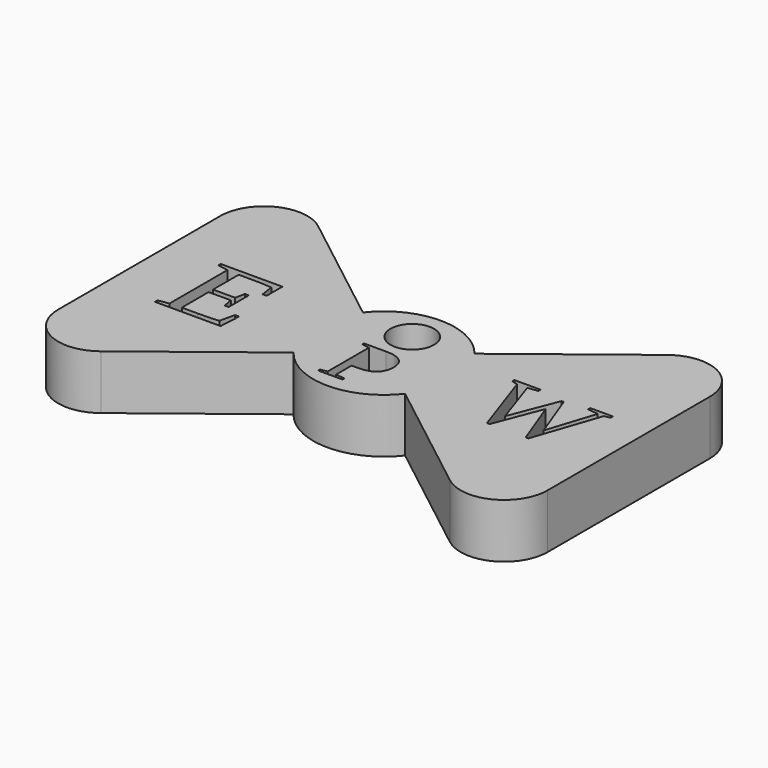
from build123d import *

# Parameters (mm, degrees)
F0_R     = 2
F1_DEPTH = 5


with BuildPart() as f1:
    # F0 (on Top) → F1 (new body)
    with BuildSketch(Plane.XY):
        with BuildLine():
            ThreePointArc((-3.8750014305, 0), (-4.2267672199, -2.1093164988), (-5.2439909973, -3.9903298027))
            Line((-5.2439909973, -3.9903298027), (5.6694109986, -12.4775612749))
            ThreePointArc((5.6694109986, -12.4775612749), (9.8825038634, -12.9132287637), (12.1249985695, -9.3200163929))
            Line((12.1249985695, -9.3200163929), (12.1249985695, 9.3200163929))
            ThreePointArc((12.1249985695, 9.3200163929), (9.8825038634, 12.9132287637), (5.6694109986, 12.4775612749))
            Line((5.6694109986, 12.4775612749), (-5.2439909973, 3.9903298027))
            ThreePointArc((-5.2439909973, 3.9903298027), (-4.2267672199, 2.1093164988), (-3.8750014305, 0))
        make_face()
        Polygon((8.0675292322, 2.2068999953), (6.0064843484, -3.8768709144), (5.756569483, -3.8768709144), (4.1200787681, 0.4710455388), (2.4399282273, -3.8768709144), (2.1900133619, -3.8768709144), (0.1018692759, 2.2068999953), (-0.449147837, 2.3288464056), (-0.449147837, 2.5787612709), (1.9596701426, 2.5787612709), (1.9596701426, 2.3288464056), (1.0337807317, 2.2068999953), (2.5347754353, -2.2388746883), (4.2329921109, 2.1361409672), (4.4437636841, 2.1361409672), (6.0817599103, -2.2388746883), (7.5119955856, 2.2068999953), (6.5288967477, 2.3288464056), (6.5288967477, 2.5787612709), (8.6170408338, 2.5787612709), (8.6170408338, 2.3288464056), align=None, mode=Mode.SUBTRACT)
        with BuildLine():
            ThreePointArc((-15.5059721811, 3.9903808286), (-16.8750014304, 3.23201e-05), (-15.5060118637, -3.9903298027))
            ThreePointArc((-15.5060118637, -3.9903298027), (-10.3750014305, -6.5), (-5.2439909973, -3.9903298027))
            ThreePointArc((-5.2439909973, -3.9903298027), (-4.2267672199, -2.1093164988), (-3.8750014305, 0))
            ThreePointArc((-3.8750014305, 0), (-4.2267672199, 2.1093164988), (-5.2439909973, 3.9903298027))
            ThreePointArc((-5.2439909973, 3.9903298027), (-10.3749691104, 6.4999999999), (-15.5059721811, 3.9903808286))
        make_face()
        with BuildLine():
            Line((-10.3772096263, -2.9674286779), (-10.9801440776, -2.9674286779))
            Line((-10.9801440776, -2.9674286779), (-10.9801440776, -4.7481291549))
            Line((-10.9801440776, -4.7481291549), (-10.1293933476, -4.8554310488))
            Line((-10.1293933476, -4.8554310488), (-10.1293933476, -5.0674800295))
            Line((-10.1293933476, -5.0674800295), (-12.385287926, -5.0674800295))
            Line((-12.385287926, -5.0674800295), (-12.385287926, -4.8554310488))
            Line((-12.385287926, -4.8554310488), (-11.7504183872, -4.7481291549))
            Line((-11.7504183872, -4.7481291549), (-11.7504183872, -0.0294006313))
            Line((-11.7504183872, -0.0294006313), (-12.4376614694, 0.0740690521))
            Line((-12.4376614694, 0.0740690521), (-12.4376614694, 0.2861180328))
            Line((-12.4376614694, 0.2861180328), (-10.4168091348, 0.2861180328))
            add(Edge.make_bspline(
                [(-10.4168091348, 0.2861180328), (-8.4534399575, 0.2861180328), (-8.4534399575, -1.2914752879)],
                knots=[0, 0, 0, 1, 1, 1], degree=2))
            add(Edge.make_bspline(
                [(-8.4534399575, -1.2914752879), (-8.4534399575, -2.1128457374), (-8.9503499185, -2.5401372077)],
                knots=[0, 0, 0, 1, 1, 1], degree=2))
            add(Edge.make_bspline(
                [(-8.9503499185, -2.5401372077), (-9.4472598794, -2.9674286779), (-10.3772096263, -2.9674286779)],
                knots=[0, 0, 0, 1, 1, 1], degree=2))
        make_face(mode=Mode.SUBTRACT)
        with Locations((-10.3750014305, 3.25)):
            Circle(F0_R, mode=Mode.SUBTRACT)
        with BuildLine():
            Line((-32.8750014305, 9.3202724501), (-32.8750014305, -9.3200163929))
            ThreePointArc((-32.8750014305, -9.3200163929), (-30.6325067245, -12.9132287637), (-26.4194138596, -12.4775612749))
            Line((-26.4194138596, -12.4775612749), (-15.5060118637, -3.9903298027))
            ThreePointArc((-15.5060118637, -3.9903298027), (-16.8750014304, 3.23201e-05), (-15.5059721811, 3.9903808286))
            Line((-15.5059721811, 3.9903808286), (-26.4193824591, 12.477792912))
            ThreePointArc((-26.4193824591, 12.477792912), (-30.6324888578, 12.9134935598), (-32.8750014305, 9.3202724501))
        make_face()
        with BuildLine():
            Line((-28.1915230864, -4.0461723693), (-28.1915230864, -3.7470318405))
            Line((-28.1915230864, -3.7470318405), (-27.2220194448, -3.5956595247))
            Line((-27.2220194448, -3.5956595247), (-27.2220194448, 3.0611182673))
            Line((-27.2220194448, 3.0611182673), (-28.1915230864, 3.2070844289))
            Line((-28.1915230864, 3.2070844289), (-28.1915230864, 3.5062249578))
            Line((-28.1915230864, 3.5062249578), (-22.5258735526, 3.5062249578))
            Line((-22.5258735526, 3.5062249578), (-22.5258735526, 1.6987674252))
            Line((-22.5258735526, 1.6987674252), (-22.8970961366, 1.6987674252))
            Line((-22.8970961366, 1.6987674252), (-23.0773012744, 2.9205582598))
            add(Edge.make_bspline(
                [(-23.0773012744, 2.9205582598), (-23.7080192569, 2.9980464691), (-24.9027793208, 2.9980464691)],
                knots=[0, 0, 0, 1, 1, 1], degree=2))
            Line((-24.9027793208, 2.9980464691), (-26.1353824636, 2.9980464691))
            Line((-26.1353824636, 2.9980464691), (-26.1353824636, 0.0480883625))
            Line((-26.1353824636, 0.0480883625), (-24.0972623546, 0.0480883625))
            Line((-24.0972623546, 0.0480883625), (-23.9224633709, 0.9491140518))
            Line((-23.9224633709, 0.9491140518), (-23.5620530952, 0.9491140518))
            Line((-23.5620530952, 0.9491140518), (-23.5620530952, -1.3719281237))
            Line((-23.5620530952, -1.3719281237), (-23.9224633709, -1.3719281237))
            Line((-23.9224633709, -1.3719281237), (-24.0972623546, -0.4582880748))
            Line((-24.0972623546, -0.4582880748), (-26.1353824636, -0.4582880748))
            Line((-26.1353824636, -0.4582880748), (-26.1353824636, -3.5397959319))
            Line((-26.1353824636, -3.5397959319), (-24.6486900764, -3.5397959319))
            add(Edge.make_bspline(
                [(-24.6486900764, -3.5397959319), (-23.1962366654, -3.5397959319), (-22.7457238208, -3.449693363)],
                knots=[0, 0, 0, 1, 1, 1], degree=2))
            Line((-22.7457238208, -3.449693363), (-22.4249586754, -2.0531035447))
            Line((-22.4249586754, -2.0531035447), (-22.0519340401, -2.0531035447))
            Line((-22.0519340401, -2.0531035447), (-22.1600571228, -4.0461723693))
            Line((-22.1600571228, -4.0461723693), (-28.1915230864, -4.0461723693))
        make_face(mode=Mode.SUBTRACT)
    extrude(amount=F1_DEPTH)


solid = f1.part
